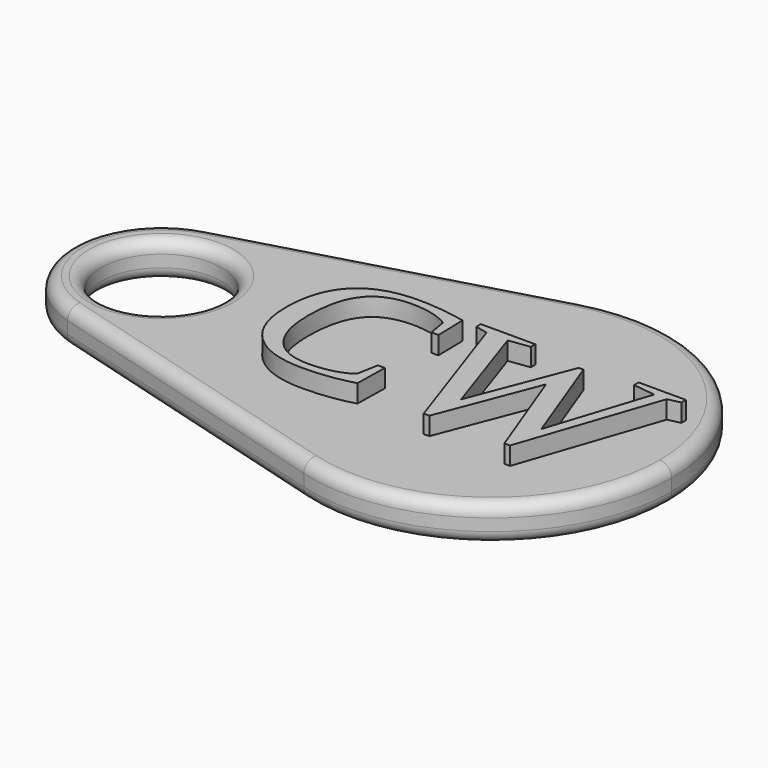
from build123d import *

# Parameters (mm, degrees)
F1_DEPTH     = 7.62
F3_R         = 12.7
F4_DEPTH     = 25.4
F2_TEXT_SIZE = 46.1149329189
F5_DEPTH     = 3.81
F6_R         = 2.54


# Not quite as in the source:
# - Text() gives the source's letters only with a copy of the font that has no kerning and outlines rounded to 1/6400 em; it was checked with that copy


with BuildPart() as f1:
    # F0 (on Top) → F1 (new body)
    with BuildSketch(Plane.XY):
        with BuildLine():
            ThreePointArc((-50.8, 0), (-58.3624177716, 15.1966428709), (-75.0454545455, 18.3278409003))
            ThreePointArc((-75.0454545455, 18.3278409003), (-88.9, 0), (-75.0454545455, -18.3278409003))
            ThreePointArc((-75.0454545455, -18.3278409003), (-58.3624177716, -15.1966428709), (-50.8, 0))
        make_face()
        with BuildLine():
            ThreePointArc((-10.3909090909, -36.6556818006), (-38.1, 0), (-10.3909090909, 36.6556818006))
            Line((-10.3909090909, 36.6556818006), (-75.0454545455, 18.3278409003))
            ThreePointArc((-75.0454545455, 18.3278409003), (-58.3624177716, 15.1966428709), (-50.8, 0))
            ThreePointArc((-50.8, 0), (-58.3624177716, -15.1966428709), (-75.0454545455, -18.3278409003))
            Line((-75.0454545455, -18.3278409003), (-10.3909090909, -36.6556818006))
        make_face()
        with BuildLine():
            ThreePointArc((-10.3909090909, -36.6556818006), (22.9751644568, -30.3932857418), (38.1, 0))
            ThreePointArc((38.1, 0), (22.9751644568, 30.3932857418), (-10.3909090909, 36.6556818006))
            ThreePointArc((-10.3909090909, 36.6556818006), (-38.1, 0), (-10.3909090909, -36.6556818006))
        make_face()
    extrude(amount=F1_DEPTH)

    # F3 (on face) → F4 (cut)
    with BuildSketch(Plane.XY.offset(7.62)):
        with Locations((-69.85, 0)):
            Circle(F3_R)
    extrude(amount=-F4_DEPTH, mode=Mode.SUBTRACT)

    # F2 (on face) → F5 (join)
    with BuildSketch(Plane.XY.offset(7.62)):
        with Locations((-44.107168606, -16.4030267218)):
            Text('CW', F2_TEXT_SIZE, font='Tinos', text_align=(TextAlign.LEFT, TextAlign.BOTTOM))
    extrude(amount=F5_DEPTH)

    # F6
    f6_edges = [f1.edges().sort_by_distance(p)[0] for p in [
        (-82.55, 0, 7.62),
        (-42.718182, -27.491761, 7.62),
        (38.1, 0, 0),
        (-82.55, 0, 0),
    ]]
    fillet(f6_edges, radius=F6_R)


solid = f1.part
